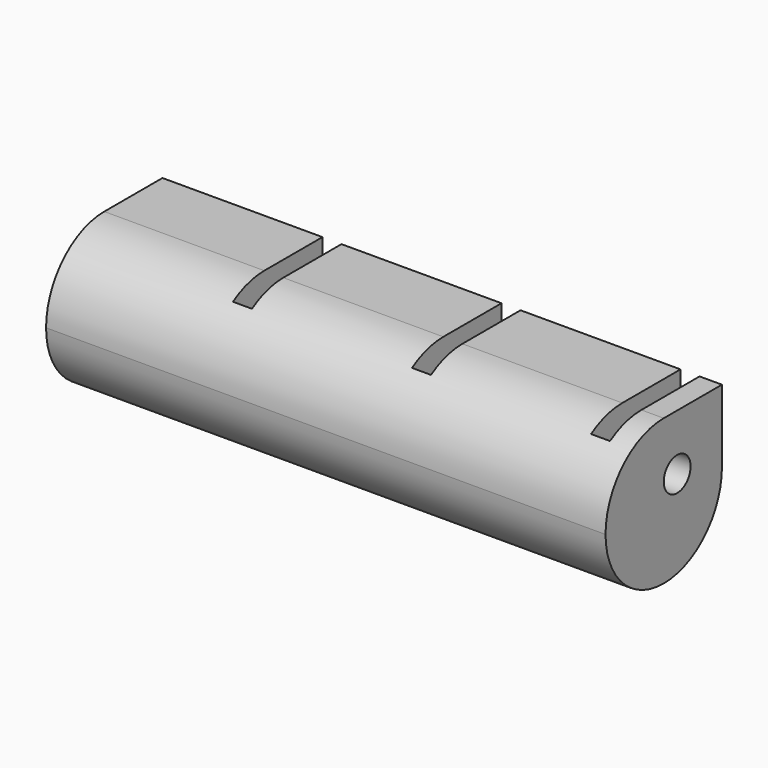
from build123d import *

# Parameters (mm, degrees)
F0_W     = 50
F0_H     = 13
F1_DEPTH = 13
F2_R     = 1.5
F3_DEPTH = 50.001
F4_R     = 6.49999
F5_W     = 1.7
F5_H     = 10
F6_DEPTH = 10


# Not quite as in the source:
# - a fillet or chamfer is up to 0.001 mm smaller than in the source, because OpenCascade refuses the exact size
# - a feature names something its author has since deleted; it is built from what else it names


with BuildPart() as f1:
    # F0 (on Top) → F1 (new body)
    with BuildSketch(Plane.XY):
        with Locations((0.8589621633, -0.6415863931)):
            Rectangle(F0_W, F0_H)
    extrude(amount=F1_DEPTH)

    # F2 (on face) → F3 (cut, through all)
    with BuildSketch(Plane.YZ.offset(25.8589621633)):
        with Locations((0.8584136069, 8)):
            Circle(F2_R)
    extrude(amount=-F3_DEPTH, mode=Mode.SUBTRACT)

    # F4 (radius 6.5 in the source; OpenCascade refuses exactly that, so slightly less here)
    f4_edges = [f1.edges().sort_by_distance(p)[0] for p in [
        (0.858962, -7.141586, 13),
        (0.858962, -7.141586, 0),
        (0.858962, 5.858414, 0),
    ]]
    fillet(f4_edges, radius=F4_R)

    # F5 (on face) → F6 (cut)
    with BuildSketch(Plane.XY.offset(13)):
        with Locations((23.0089621633, 0.8584136069)):
            Rectangle(F5_W, F5_H)
        with Locations((7.0089621633, 0.8584136069)):
            Rectangle(F5_W, F5_H)
        with Locations((-8.9910378367, 0.8584136069)):
            Rectangle(F5_W, F5_H)
    extrude(amount=-F6_DEPTH, mode=Mode.SUBTRACT)


solid = f1.part
